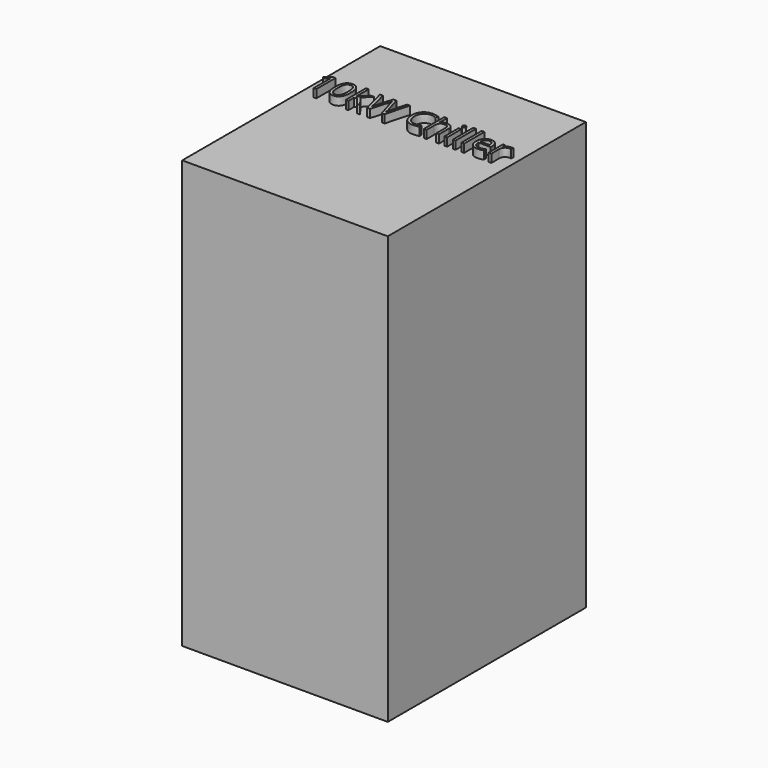
from build123d import *

# Parameters (mm, degrees)
F0_W         = 638.175
F0_H         = 768.35
F1_DEPTH     = 1327.15
F2_TEXT_SIZE = 103.7175669928
F3_DEPTH     = 25.4


# Not quite as in the source:
# - Text() gives the source's letters only with a copy of the font that has no kerning and outlines rounded to 1/6400 em; it was checked with that copy


with BuildPart() as f1:
    # F0 (on Top) → F1 (new body)
    with BuildSketch(Plane.XY):
        Rectangle(F0_W, F0_H)
    extrude(amount=F1_DEPTH)

    # F2 (on face) → F3 (join)
    with BuildSketch(Plane.XY.offset(1327.15)):
        with Locations((-304.8, 73.2142613359)):
            Text('10kW Chiller', F2_TEXT_SIZE, font='Open Sans', text_align=(TextAlign.LEFT, TextAlign.BOTTOM))
    extrude(amount=F3_DEPTH)


solid = f1.part
